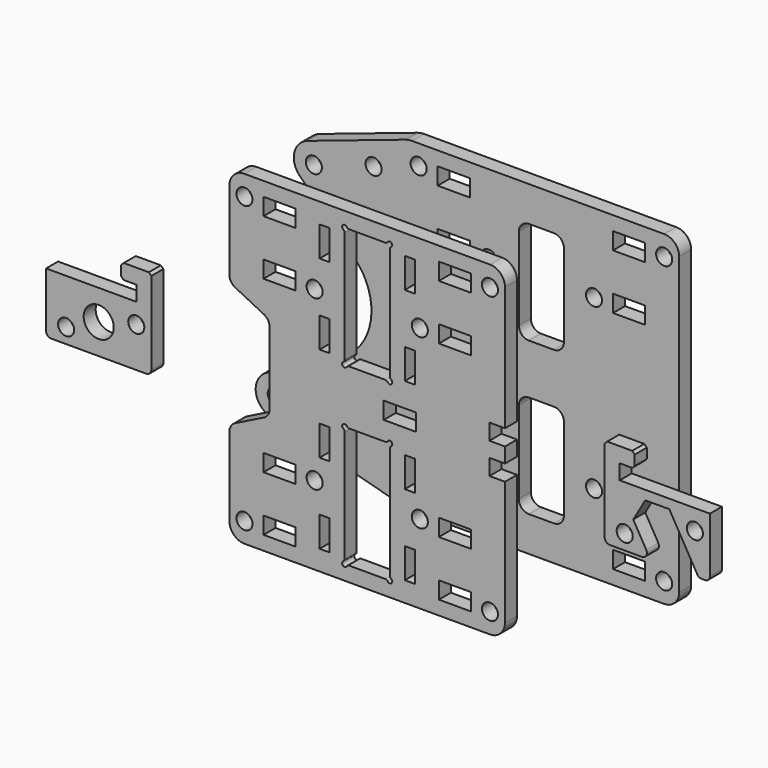
from build123d import *

# Parameters (mm, degrees)
F0_R      = 1.6
F0_W      = 6.4
F0_H      = 3.4
F0_W_2    = 2
F0_H_2    = 6
F1_DEPTH  = 3
F3_R      = 1.60312
F3_W      = 6.4
F3_H      = 3.4
F3_R_2    = 1.6
F4_DEPTH  = 3
F11_R     = 1.60312
F12_DEPTH = 3
F11_R_2   = 3


# Not quite as in the source:
# - ends of sketch curves that miss each other by under 0.0002 mm in the source are joined


with BuildPart() as f1:
    # F0 (on Front) → F1 (new body)
    with BuildSketch(Plane.XZ):
        with BuildLine():
            Line((27.5, -1.5), (27.5, 1.5))
            Line((27.5, 1.5), (24.4, 1.5))
            Line((24.4, 1.5), (24.4, 4.7))
            Line((24.4, 4.7), (27.5, 4.7))
            Line((27.5, 4.7), (27.5, 29.5))
            ThreePointArc((27.5, 29.5), (26.6213203436, 31.6213203436), (24.5, 32.5))
            Line((24.5, 32.5), (-24.5, 32.5))
            ThreePointArc((-24.5, 32.5), (-26.6213203436, 31.6213203436), (-27.5, 29.5))
            Line((-27.5, 29.5), (-27.5, 13.736068))
            ThreePointArc((-27.5, 13.736068), (-27.2013016167, 12.6846057758), (-26.394427191, 11.947213618))
            Line((-26.394427191, 11.947213618), (-20.605573, 9.052786))
            ThreePointArc((-20.605573, 9.052786), (-19.7986983833, 8.3153942242), (-19.5, 7.263932))
            Line((-19.5, 7.263932), (-19.5, -7.263932))
            ThreePointArc((-19.5, -7.263932), (-19.7986983833, -8.3153942242), (-20.605572809, -9.052786382))
            Line((-20.605572809, -9.052786382), (-26.394427, -11.947214))
            ThreePointArc((-26.394427, -11.947214), (-27.2013016167, -12.6846057758), (-27.5, -13.736068))
            Line((-27.5, -13.736068), (-27.5, -29.5))
            ThreePointArc((-27.5, -29.5), (-26.6213203436, -31.6213203436), (-24.5, -32.5))
            Line((-24.5, -32.5), (24.5, -32.5))
            ThreePointArc((24.5, -32.5), (26.6213203436, -31.6213203436), (27.5, -29.5))
            Line((27.5, -29.5), (27.5, -4.7))
            Line((27.5, -4.7), (24.4, -4.7))
            Line((24.4, -4.7), (24.4, -1.5))
            Line((24.4, -1.5), (27.5, -1.5))
        make_face()
        with Locations((-24.5, -28.5)):
            Circle(F0_R, mode=Mode.SUBTRACT)
        with Locations((-17.5, -28)):
            Rectangle(F0_W, F0_H, mode=Mode.SUBTRACT)
        with Locations((-17.5, -17)):
            Rectangle(F0_W, F0_H, mode=Mode.SUBTRACT)
        with Locations((-8.5, -25.5)):
            Rectangle(F0_W_2, F0_H_2, mode=Mode.SUBTRACT)
        with Locations((-10.5, -16.8)):
            Circle(F0_R, mode=Mode.SUBTRACT)
        with Locations((-8.5, -9.5)):
            Rectangle(F0_W_2, F0_H_2, mode=Mode.SUBTRACT)
        with Locations((8.5, -25.5)):
            Rectangle(F0_W_2, F0_H_2, mode=Mode.SUBTRACT)
        with BuildLine():
            ThreePointArc((4.0669972236, -5.1999901291), (4.8535627309, -5.0964359497), (4.7500114869, -5.8830018434))
            ThreePointArc((4.7500114869, -5.8830018434), (4.5669973354, -6.0660199355), (4.50001, -6.31602))
            Line((4.50001, -6.31602), (4.50001, -28.683999))
            ThreePointArc((4.50001, -28.683999), (4.5669973354, -28.9339990645), (4.7500101291, -29.1170117764))
            ThreePointArc((4.7500101291, -29.1170117764), (4.8535632138, -29.9035525674), (4.0669972236, -29.7999988709))
            ThreePointArc((4.0669972236, -29.7999988709), (3.8840100645, -29.6169863354), (3.63401, -29.549999))
            Line((3.63401, -29.549999), (-3.63399, -29.549999))
            ThreePointArc((-3.63399, -29.549999), (-3.8839900645, -29.6169863354), (-4.0670027764, -29.7999991291))
            ThreePointArc((-4.0670027764, -29.7999991291), (-4.853544003, -29.9035517782), (-4.7499903039, -29.1169864736))
            ThreePointArc((-4.7499903039, -29.1169864736), (-4.5669773354, -28.9339990645), (-4.49999, -28.683999))
            Line((-4.49999, -28.683999), (-4.49999, -6.316029))
            ThreePointArc((-4.49999, -6.316029), (-4.5669772104, -6.066029152), (-4.7499896961, -5.8830164736))
            ThreePointArc((-4.7499896961, -5.8830164736), (-4.8535433906, -5.0964456094), (-4.0669772236, -5.1999991291))
            ThreePointArc((-4.0669772236, -5.1999991291), (-3.8839900645, -5.3830116646), (-3.63399, -5.449999))
            Line((-3.63399, -5.449999), (3.63401, -5.44999))
            ThreePointArc((3.63401, -5.44999), (3.8840100645, -5.3830026646), (4.0669972236, -5.1999901291))
        make_face(mode=Mode.SUBTRACT)
        with Locations((10.5, -16.8)):
            Circle(F0_R, mode=Mode.SUBTRACT)
        with Locations((17.5, -28)):
            Rectangle(F0_W, F0_H, mode=Mode.SUBTRACT)
        with Locations((24.5, -28.5)):
            Circle(F0_R, mode=Mode.SUBTRACT)
        with Locations((17.5, -17)):
            Rectangle(F0_W, F0_H, mode=Mode.SUBTRACT)
        with Locations((8.5, -9.5)):
            Rectangle(F0_W_2, F0_H_2, mode=Mode.SUBTRACT)
        with Locations((-8.5, 9.5)):
            Rectangle(F0_W_2, F0_H_2, mode=Mode.SUBTRACT)
        with Locations((-17.5, 17)):
            Rectangle(F0_W, F0_H, mode=Mode.SUBTRACT)
        with Locations((-24.5, 28.5)):
            Circle(F0_R, mode=Mode.SUBTRACT)
        with Locations((-17.5, 28)):
            Rectangle(F0_W, F0_H, mode=Mode.SUBTRACT)
        with Locations((-10.5, 16.8)):
            Circle(F0_R, mode=Mode.SUBTRACT)
        with Locations((-8.5, 25.5)):
            Rectangle(F0_W_2, F0_H_2, mode=Mode.SUBTRACT)
        with Locations((6.5, 0)):
            Rectangle(F0_W, F0_H, mode=Mode.SUBTRACT)
        with Locations((8.5, 9.5)):
            Rectangle(F0_W_2, F0_H_2, mode=Mode.SUBTRACT)
        with BuildLine():
            ThreePointArc((4.0669972236, 29.8000098709), (4.8535627309, 29.9035640503), (4.7500114869, 29.1169981566))
            ThreePointArc((4.7500114869, 29.1169981566), (4.5669972104, 28.933980848), (4.50001, 28.683981))
            Line((4.50001, 28.683981), (4.50001, 6.316001))
            ThreePointArc((4.50001, 6.316001), (4.5669973354, 6.0660009355), (4.7500101291, 5.8829882236))
            ThreePointArc((4.7500101291, 5.8829882236), (4.8535633906, 5.0964466094), (4.0669972236, 5.2000001291))
            ThreePointArc((4.0669972236, 5.2000001291), (3.8840100645, 5.3830126646), (3.63401, 5.45))
            Line((3.63401, 5.45), (-3.63399, 5.45))
            ThreePointArc((-3.63399, 5.45), (-3.8839900645, 5.3830126646), (-4.0670027764, 5.1999998709))
            ThreePointArc((-4.0670027764, 5.1999998709), (-4.8535438736, 5.0964470924), (-4.7499898709, 5.8830127764))
            ThreePointArc((-4.7499898709, 5.8830127764), (-4.5669773354, 6.0660009355), (-4.49999, 6.316001))
            Line((-4.49999, 6.316001), (-4.49999, 28.683971))
            ThreePointArc((-4.49999, 28.683971), (-4.5669772104, 28.933970848), (-4.7499896961, 29.1169835264))
            ThreePointArc((-4.7499896961, 29.1169835264), (-4.8535432138, 29.9035535674), (-4.0669772236, 29.7999998709))
            ThreePointArc((-4.0669772236, 29.7999998709), (-3.8839900645, 29.6169873354), (-3.63399, 29.55))
            Line((-3.63399, 29.55), (3.63401, 29.55001))
            ThreePointArc((3.63401, 29.55001), (3.8840100645, 29.6169973354), (4.0669972236, 29.8000098709))
        make_face(mode=Mode.SUBTRACT)
        with Locations((10.5, 16.8)):
            Circle(F0_R, mode=Mode.SUBTRACT)
        with Locations((8.5, 25.5)):
            Rectangle(F0_W_2, F0_H_2, mode=Mode.SUBTRACT)
        with Locations((17.5, 17)):
            Rectangle(F0_W, F0_H, mode=Mode.SUBTRACT)
        with Locations((17.5, 28)):
            Rectangle(F0_W, F0_H, mode=Mode.SUBTRACT)
        with Locations((24.5, 28.5)):
            Circle(F0_R, mode=Mode.SUBTRACT)
    extrude(amount=F1_DEPTH)


with BuildPart() as f4:
    # F3 (on offset) → F4 (new body)
    with BuildSketch(Plane.XZ.offset(-25)):
        with BuildLine():
            ThreePointArc((-31.9281980521, 25.7118451549), (-34.5478832539, 22.8344181994), (-33.4821601247, 19.0918828753))
            Line((-33.4821601247, 19.0918828753), (-22.522005, 8.131728))
            ThreePointArc((-22.522005, 8.131728), (-19.2963295887, -1.8053774543), (-25.4443590177, -10.2524349651))
            Line((-25.4443590177, -10.2524349651), (-40.078533, -17.688218))
            ThreePointArc((-40.078533, -17.688218), (-42.2448641745, -21.6704924723), (-39.3012089638, -25.1181578649))
            Line((-39.3012089638, -25.1181578649), (-12.241784, -32.363876))
            ThreePointArc((-12.241784, -32.363876), (-11.7289261563, -32.4658229574), (-11.207152, -32.5))
            Line((-11.207152, -32.5), (39.266577, -32.5))
            ThreePointArc((39.266577, -32.5), (41.3878973436, -31.6213203436), (42.266577, -29.5))
            Line((42.266577, -29.5), (42.266577, 29.5))
            ThreePointArc((42.266577, 29.5), (41.3878973436, 31.6213203436), (39.266577, 32.5))
            Line((39.266577, 32.5), (-11.079141, 32.5))
            ThreePointArc((-11.079141, 32.5), (-11.7248419293, 32.4475397794), (-12.3536060521, 32.2915351549))
            Line((-12.3536060521, 32.2915351549), (-31.9281980521, 25.7118451549))
        make_face()
        with BuildLine():
            ThreePointArc((-38.5444139008, -22.8299744372), (-39.8422694221, -20.9764450137), (-37.9887399282, -19.678589593))
            ThreePointArc((-37.9887399282, -19.678589593), (-34.3352457699, -20.1595816741), (-30.653733, -20.32032))
            ThreePointArc((-30.653733, -20.32032), (-29.053733, -21.9203), (-30.653733, -23.5203))
            ThreePointArc((-30.653733, -23.5203), (-34.6141440475, -23.3474047167), (-38.5444139008, -22.8299744372))
        make_face(mode=Mode.SUBTRACT)
        with Locations((-9.733423, -28.5)):
            Circle(F3_R, mode=Mode.SUBTRACT)
        with Locations((-2.733423, -28)):
            Rectangle(F3_W, F3_H, mode=Mode.SUBTRACT)
        with Locations((-2.733423, -17)):
            Rectangle(F3_W, F3_H, mode=Mode.SUBTRACT)
        with BuildLine():
            ThreePointArc((-9.8647938499, 1.1313708499), (-7.6020521501, 1.1313708499), (-7.6020521501, -1.1313708499))
            ThreePointArc((-7.6020521501, -1.1313708499), (-9.6988569476, -3.0527488653), (-11.9551412249, -4.7840566788))
            ThreePointArc((-11.9551412249, -4.7840566788), (-14.1835062514, -4.3911353259), (-13.7905858964, -2.162770148))
            ThreePointArc((-13.7905858964, -2.162770148), (-11.7557773245, -0.6014066691), (-9.8647938499, 1.1313708499))
        make_face(mode=Mode.SUBTRACT)
        with Locations((4.266577, -16.8)):
            Circle(F3_R_2, mode=Mode.SUBTRACT)
        with Locations((39.266577, -28.5)):
            Circle(F3_R, mode=Mode.SUBTRACT)
        with Locations((32.266577, -28)):
            Rectangle(F3_W, F3_H, mode=Mode.SUBTRACT)
        with Locations((25.266577, -16.8)):
            Circle(F3_R_2, mode=Mode.SUBTRACT)
        with Locations((32.266577, -17)):
            Rectangle(F3_W, F3_H, mode=Mode.SUBTRACT)
        with BuildLine():
            ThreePointArc((19.266577, -23.5), (18.6807905624, -24.9142135624), (17.266577, -25.5))
            Line((17.266577, -25.5), (12.266577, -25.5))
            ThreePointArc((12.266577, -25.5), (10.8523634376, -24.9142135624), (10.266577, -23.5))
            Line((10.266577, -23.5), (10.266577, -7))
            ThreePointArc((10.266577, -7), (10.8523634376, -5.5857864376), (12.266577, -5))
            Line((12.266577, -5), (17.266577, -5))
            ThreePointArc((17.266577, -5), (18.6807905624, -5.5857864376), (19.266577, -7))
            Line((19.266577, -7), (19.266577, -23.5))
        make_face(mode=Mode.SUBTRACT)
        with Locations((-30.653733, 21.92031)):
            Circle(F3_R, mode=Mode.SUBTRACT)
        with Locations((-2.733423, 17)):
            Rectangle(F3_W, F3_H, mode=Mode.SUBTRACT)
        with Locations((-18.733423, 25.5)):
            Circle(F3_R, mode=Mode.SUBTRACT)
        with Locations((-2.733423, 28)):
            Rectangle(F3_W, F3_H, mode=Mode.SUBTRACT)
        with Locations((-9.733423, 28.5)):
            Circle(F3_R, mode=Mode.SUBTRACT)
        with BuildLine():
            ThreePointArc((17.266577, 25.5), (18.6807905624, 24.9142135624), (19.266577, 23.5))
            Line((19.266577, 23.5), (19.266577, 7))
            ThreePointArc((19.266577, 7), (18.6807905624, 5.5857864376), (17.266577, 5))
            Line((17.266577, 5), (12.266577, 5))
            ThreePointArc((12.266577, 5), (10.8523634376, 5.5857864376), (10.266577, 7))
            Line((10.266577, 7), (10.266577, 23.5))
            ThreePointArc((10.266577, 23.5), (10.8523634376, 24.9142135624), (12.266577, 25.5))
            Line((12.266577, 25.5), (17.266577, 25.5))
        make_face(mode=Mode.SUBTRACT)
        with Locations((4.266577, 16.8)):
            Circle(F3_R_2, mode=Mode.SUBTRACT)
        with Locations((25.266577, 16.8)):
            Circle(F3_R_2, mode=Mode.SUBTRACT)
        with Locations((32.266577, 17)):
            Rectangle(F3_W, F3_H, mode=Mode.SUBTRACT)
        with Locations((32.266577, 28)):
            Rectangle(F3_W, F3_H, mode=Mode.SUBTRACT)
        with Locations((39.266577, 28.5)):
            Circle(F3_R, mode=Mode.SUBTRACT)
    extrude(amount=F4_DEPTH)


with BuildPart() as f12:
    # F11 (on Front) → F12 (new body)
    with BuildSketch(Plane.XZ):
        with BuildLine():
            Line((68.3999997377, 3.0000003874), (50.3999997377, 3.0000003874))
            Line((50.3999997377, 3.0000003874), (50.3999997377, 6.0000003874))
            Line((50.3999997377, 6.0000003874), (52.8999997377, 6.0000003874))
            Line((52.8999997377, 6.0000003874), (53.3999997377, 6.5000003874))
            Line((53.3999997377, 6.5000003874), (53.3999997377, 8.5000003874))
            Line((53.3999997377, 8.5000003874), (52.8999997377, 9.0000003874))
            Line((52.8999997377, 9.0000003874), (47.8999997377, 9.0000003874))
            Line((47.8999997377, 9.0000003874), (47.3999997377, 8.5000003874))
            Line((47.3999997377, 8.5000003874), (47.3999997377, -7.9999996126))
            ThreePointArc((47.3999997377, -7.9999996126), (47.6928929566, -8.7071063938), (48.3999997377, -8.9999996126))
            Line((48.3999997377, -8.9999996126), (54.8319747377, -8.9999996126))
            ThreePointArc((54.8319747377, -8.9999996126), (55.6979970604, -8.5000049492), (55.6980063037, -7.5000102858))
            Line((55.6980063037, -7.5000102858), (53.0999997377, -2.9999996126))
            Line((53.0999997377, -2.9999996126), (55.4999997377, 1.1569223874))
            Line((55.4999997377, 1.1569223874), (60.2999997377, 1.1569223874))
            Line((60.2999997377, 1.1569223874), (65.8754257377, -8.4999996126))
            ThreePointArc((65.8754257377, -8.4999996126), (66.2414516087, -8.8660249418), (66.7414517377, -8.9999996126))
            Line((66.7414517377, -8.9999996126), (67.3999997377, -8.9999996126))
            ThreePointArc((67.3999997377, -8.9999996126), (68.1071065189, -8.7071063938), (68.3999997377, -7.9999996126))
            Line((68.3999997377, -7.9999996126), (68.3999997377, 3.0000003874))
        make_face()
        with Locations((51.3999997377, -5.9999996126)):
            Circle(F11_R, mode=Mode.SUBTRACT)
        with Locations((65.3999997377, -0.9999996126)):
            Circle(F11_R, mode=Mode.SUBTRACT)
    extrude(amount=F12_DEPTH)


with BuildPart() as f12b:
    # F11 (on Front) → F12, piece 2 (new body)
    with BuildSketch(Plane.XZ):
        with BuildLine():
            Line((-48.6000101566, 6.0000003874), (-46.1000101566, 6.0000003874))
            Line((-46.1000101566, 6.0000003874), (-46.1000101566, 3.0000003874))
            Line((-46.1000101566, 3.0000003874), (-64.1000101566, 3.0000003874))
            Line((-64.1000101566, 3.0000003874), (-64.1000101566, -7.9999996126))
            ThreePointArc((-64.1000101566, -7.9999996126), (-63.8071169378, -8.7071063938), (-63.1000101566, -8.9999996126))
            Line((-63.1000101566, -8.9999996126), (-44.1000101566, -8.9999996126))
            ThreePointArc((-44.1000101566, -8.9999996126), (-43.3929033754, -8.7071063938), (-43.1000101566, -7.9999996126))
            Line((-43.1000101566, -7.9999996126), (-43.1000101566, 8.5000003874))
            Line((-43.1000101566, 8.5000003874), (-43.6000101566, 9.0000003874))
            Line((-43.6000101566, 9.0000003874), (-48.6000101566, 9.0000003874))
            Line((-48.6000101566, 9.0000003874), (-49.1000101566, 8.5000003874))
            Line((-49.1000101566, 8.5000003874), (-49.1000101566, 6.5000003874))
            Line((-49.1000101566, 6.5000003874), (-48.6000101566, 6.0000003874))
        make_face()
        with Locations((-60.1000101566, -5.9999996126)):
            Circle(F11_R, mode=Mode.SUBTRACT)
        with Locations((-53.6000101566, -2.9999996126)):
            Circle(F11_R_2, mode=Mode.SUBTRACT)
        with Locations((-46.1000101566, -0.9999996126)):
            Circle(F11_R, mode=Mode.SUBTRACT)
    extrude(amount=F12_DEPTH)


solid = Compound([f1.part, f4.part, f12.part, f12b.part])
